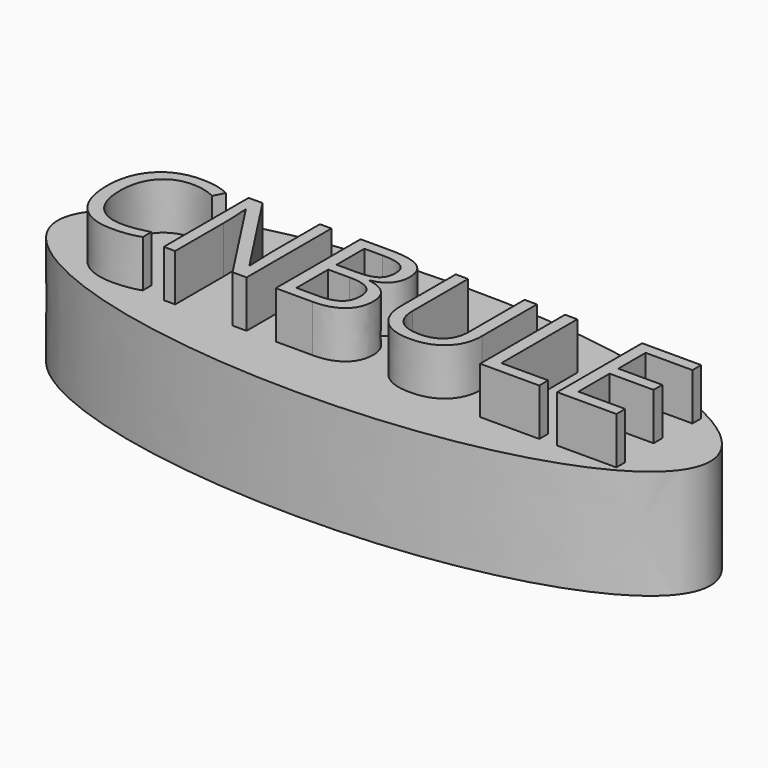
from build123d import *

# Parameters (mm, degrees)
F1_DEPTH     = 25.4
F2_TEXT_SIZE = 34.5067590027
F3_DEPTH     = 10.922


# Not quite as in the source:
# - Text() gives the source's letters only with a copy of the font that has no kerning and outlines rounded to 1/6400 em; it was checked with that copy


with BuildPart() as f1:
    # F0 (on Top) → F1 (new body)
    with BuildSketch(Plane.XY):
        with BuildLine():
            add(Edge.make_bspline(
                [(75.7867917418, 0), (75.7867917418, 44.3418078765), (-37.8933958709, 22.1709039382), (-151.5735834837, 0), (-37.8933958709, -22.1709039382), (75.7867917418, -44.3418078765), (75.7867917418, 0)],
                knots=[0, 0, 0, 2.0943951024, 2.0943951024, 4.1887902048, 4.1887902048, 6.2831853072, 6.2831853072, 6.2831853072], degree=2, weights=[1, 0.5, 1, 0.5, 1, 0.5, 1]))
        make_face()
    extrude(amount=F1_DEPTH)

    # F2 (on face) → F3 (join)
    with BuildSketch(Plane.XY.offset(25.4)):
        with Locations((-66.345678733, -12.4706560732)):
            Text('CNBULE', F2_TEXT_SIZE, font='Open Sans', text_align=(TextAlign.LEFT, TextAlign.BOTTOM))
    extrude(amount=F3_DEPTH)


solid = f1.part
